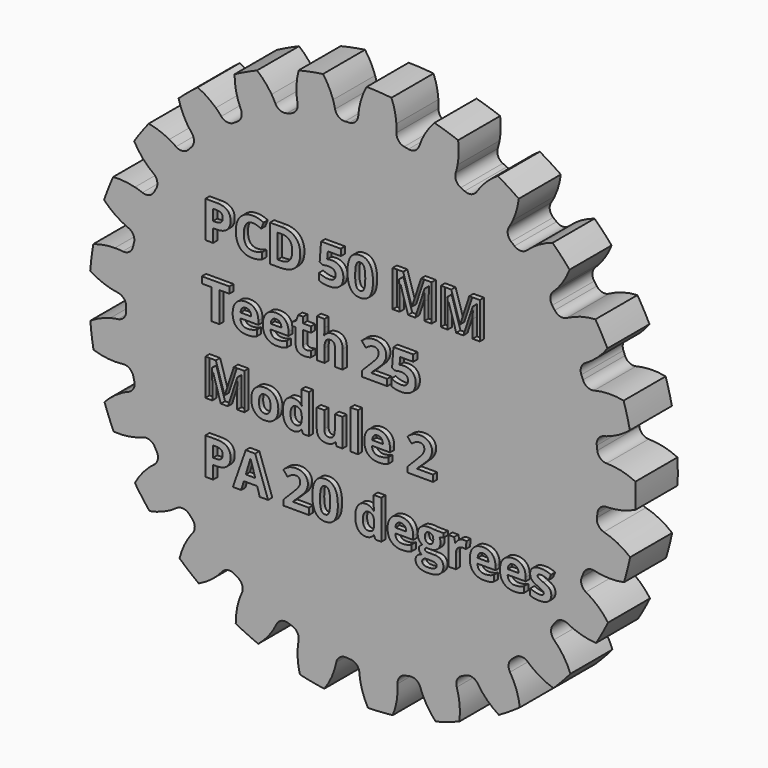
from build123d import *

# Parameters (mm, degrees)
F1_DEPTH     = 5
F2_R         = 0.897959184
F3_COUNT     = 25
F4_TEXT_SIZE = 4.8611111111
F5_DEPTH     = 0.5


# Not quite as in the source:
# - Text() gives the source's letters only with a copy of the font that has no kerning and outlines rounded to 1/6400 em; it was checked with that copy


with BuildPart() as f1:
    # F0 (on Front) → F1 (new body)
    with BuildSketch(Plane.XZ):
        with BuildLine():
            ThreePointArc((2.7489771662, 25.854267047), (1.5713354453, 25.9524739653), (0.3904476507, 25.9970681161))
            ThreePointArc((0.3904476507, 25.9970681161), (-0.2634161981, 24.3041173902), (-0.4202655523, 22.4960746991))
            ThreePointArc((-0.4202655523, 22.4960746991), (-1.35980952, -22.4588717007), (3.1313696965, 22.2810350708))
            ThreePointArc((3.1313696965, 22.2810350708), (3.2206794389, 23.0525561088), (3.2166946834, 23.8292188825))
            ThreePointArc((3.2166946834, 23.8292188825), (3.0648607141, 24.8606879121), (2.7489771662, 25.854267047))
        make_face()
    extrude(amount=F1_DEPTH)

    # F2
    f2_edges = [f1.edges().sort_by_distance(p)[0] for p in [
        (-0.420266, -2.5, 22.496075),
        (3.13137, -2.5, 22.281035),
    ]]
    fillet(f2_edges, radius=F2_R)

    # F3: F1 ×25 about axis
    f3_axis = Axis((0, 0, 0), (0, 1, 0))


with BuildPart() as f1_1:
    add(f1.part)
    for i in range(1, F3_COUNT):
        add(f1.part.rotate(f3_axis, i * 360 / F3_COUNT))

    # F4 (on face) → F5 (join)
    with BuildSketch(Plane.XZ.offset(5)):
        with Locations((-15, 8.5)):
            Text('PCD 50 MM', F4_TEXT_SIZE, font='Open Sans', font_style=FontStyle.BOLD, text_align=(TextAlign.LEFT, TextAlign.BOTTOM))
        with Locations((-15, 1.8888888889)):
            Text('Teeth 25', F4_TEXT_SIZE, font='Open Sans', font_style=FontStyle.BOLD, text_align=(TextAlign.LEFT, TextAlign.BOTTOM))
        with Locations((-15, -4.7222222222)):
            Text('Module 2', F4_TEXT_SIZE, font='Open Sans', font_style=FontStyle.BOLD, text_align=(TextAlign.LEFT, TextAlign.BOTTOM))
        with Locations((-15, -11.3333333333)):
            Text('PA 20 degrees', F4_TEXT_SIZE, font='Open Sans', font_style=FontStyle.BOLD, text_align=(TextAlign.LEFT, TextAlign.BOTTOM))
    extrude(amount=F5_DEPTH)


solid = f1_1.part
